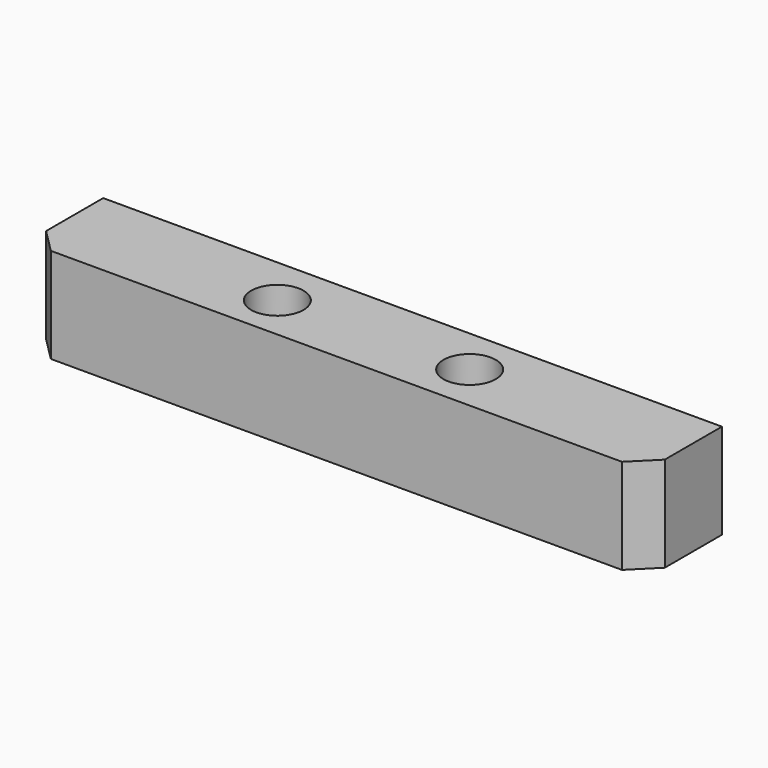
from build123d import *

# Parameters (mm, degrees)
F0_R     = 5.5
F2_DEPTH = 20
F4_D     = 5.5
F4_DEPTH = 12
F4_TIP   = 1.6523667023


# Not quite as in the source:
# - the program builds the solid bodies; features that only make, move or delete a surface that nothing else refers to are left out


with BuildPart() as f2:
    # F0 (on Top) → F2 (new body)
    with BuildSketch(Plane.XY):
        Polygon((64.6278701635, 0.2722779787), (-65.3721298365, 0.2722779787), (-65.3721298365, -14.7277220213), (-60.3721298365, -19.7277220213), (59.6278701635, -19.7277220213), (64.6278701635, -14.7314790532), align=None)
        with Locations((-20.3721298365, -10.2438455071)):
            Circle(F0_R, mode=Mode.SUBTRACT)
        with Locations((19.6245402317, -9.7277220213)):
            Circle(F0_R, mode=Mode.SUBTRACT)
    extrude(amount=F2_DEPTH)

    # F4 (one way)
    with BuildSketch(Plane.XZ):
        with Locations((0, 15)):
            Circle(F4_D / 2)
    extrude(amount=-F4_DEPTH, mode=Mode.SUBTRACT)
    with Locations(Plane.XZ):
        with Locations((0, 15)):
            with Locations((0, 0, -(F4_DEPTH + F4_TIP / 2))):  # 118° drill point
                Cone(0, F4_D / 2, F4_TIP, mode=Mode.SUBTRACT)


solid = f2.part
